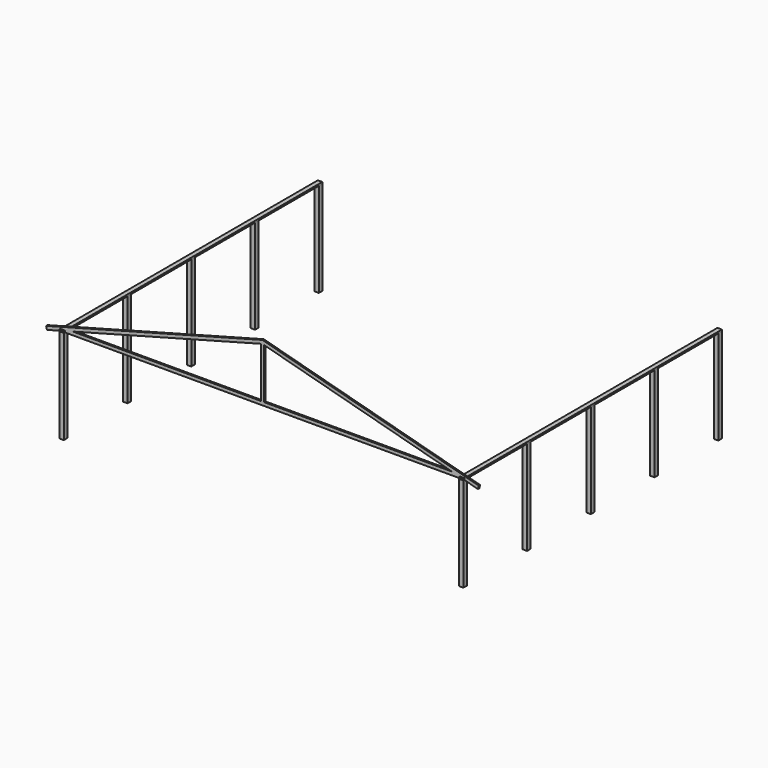
from build123d import *

# Parameters (mm, degrees)
F5_W      = 101.6
F5_H      = 101.6
F6_DEPTH  = 2133.6
F7_T      = -3.048
F7_2_T    = -3.048
F7_3_T    = -3.048
F7_4_T    = -3.048
F7_5_T    = -3.048
F11_DEPTH = 19.05
F10_W     = 76.2
F10_H     = 76.2
F12_DEPTH = 19.05
F13_T     = -3.048
F14_W     = 101.6
F14_H     = 38.1
F15_DEPTH = 7315.2
F16_T     = -3.048


with BuildPart() as f6:
    # F5 (on Top) → F6 (new body)
    with BuildSketch(Plane.XY):
        with Locations((-4521.2, 3606.8)):
            Rectangle(F5_W, F5_H)
    extrude(amount=F6_DEPTH)

    # F7
    f7_openings = [f6.faces().sort_by_distance(p)[0] for p in [
        (-4521.2, 3606.8, 2133.6),
        (-4521.2, 3606.8, 0),
    ]]
    offset(amount=F7_T, openings=f7_openings)


with BuildPart() as f6b:
    # F5 (on Top) → F6, piece 2 (new body)
    with BuildSketch(Plane.XY):
        with Locations((-4521.2, 1803.4)):
            Rectangle(F5_W, F5_H)
    extrude(amount=F6_DEPTH)

    # F7#2
    f7_2_openings = [f6b.faces().sort_by_distance(p)[0] for p in [
        (-4521.2, 1803.4, 2133.6),
        (-4521.2, 1803.4, 0),
    ]]
    offset(amount=F7_2_T, openings=f7_2_openings)


with BuildPart() as f6c:
    # F5 (on Top) → F6, piece 3 (new body)
    with BuildSketch(Plane.XY):
        with Locations((-4521.2, 0)):
            Rectangle(F5_W, F5_H)
    extrude(amount=F6_DEPTH)

    # F7#3
    f7_3_openings = [f6c.faces().sort_by_distance(p)[0] for p in [
        (-4521.2, 0, 2133.6),
        (-4521.2, 0, 0),
    ]]
    offset(amount=F7_3_T, openings=f7_3_openings)


with BuildPart() as f6d:
    # F5 (on Top) → F6, piece 4 (new body)
    with BuildSketch(Plane.XY):
        with Locations((-4521.2, -1803.4)):
            Rectangle(F5_W, F5_H)
    extrude(amount=F6_DEPTH)

    # F7#4
    f7_4_openings = [f6d.faces().sort_by_distance(p)[0] for p in [
        (-4521.2, -1803.4, 2133.6),
        (-4521.2, -1803.4, 0),
    ]]
    offset(amount=F7_4_T, openings=f7_4_openings)


with BuildPart() as f6e:
    # F5 (on Top) → F6, piece 5 (new body)
    with BuildSketch(Plane.XY):
        with Locations((-4521.2, -3606.8)):
            Rectangle(F5_W, F5_H)
    extrude(amount=F6_DEPTH)

    # F7#5
    f7_5_openings = [f6e.faces().sort_by_distance(p)[0] for p in [
        (-4521.2, -3606.8, 2133.6),
        (-4521.2, -3606.8, 0),
    ]]
    offset(amount=F7_5_T, openings=f7_5_openings)


with BuildPart() as f8_1:
    # F8: instance of F6c
    add(f6c.part.mirror(Plane.YZ))


with BuildPart() as f8_2:
    # F8: instance of F6d
    add(f6d.part.mirror(Plane.YZ))


with BuildPart() as f8_3:
    # F8: instance of F6e
    add(f6e.part.mirror(Plane.YZ))


with BuildPart() as f8_4:
    # F8: instance of F6b
    add(f6b.part.mirror(Plane.YZ))


with BuildPart() as f8_5:
    # F8: instance of F6
    add(f6.part.mirror(Plane.YZ))


with BuildPart() as f11:
    # F10 (on mid) → F11 (new body, symmetric)
    with BuildSketch(Plane.XZ.offset(3606.8)):
        Polygon((-4572, 2133.6), (-4572, 2209.8), (-4287.6177284633, 2209.8), (-38.1, 3348.4548435635), (0, 3358.6637077951), (38.1, 3348.4548435635), (4287.6177284633, 2209.8), (4572, 2209.8), (4572, 2133.6), (4876.8, 2051.929086147), (4896.5220112368, 2125.5326341102), (0, 3437.5517527423), (-4896.5220112368, 2125.5326341102), (-4876.8, 2051.929086147), align=None)
        Polygon((-4287.6177284633, 2209.8), (-4572, 2209.8), (-4572, 2133.6), align=None)
        Polygon((4572, 2209.8), (4287.6177284633, 2209.8), (4572, 2133.6), align=None)
    extrude(amount=F11_DEPTH, both=True)

    # F10 (on mid) → F12 (join, symmetric)
    with BuildSketch(Plane.XZ.offset(3606.8)):
        Polygon((-38.1, 2209.8), (-4287.6177284633, 2209.8), (-4572, 2133.6), (-38.1, 2133.6), align=None)
        Polygon((4287.6177284633, 2209.8), (38.1, 2209.8), (38.1, 2133.6), (4572, 2133.6), align=None)
        with Locations((0, 2171.7)):
            Rectangle(F10_W, F10_H)
        Polygon((-38.1, 3348.4548435635), (-38.1, 2209.8), (38.1, 2209.8), (38.1, 3348.4548435635), (0, 3358.6637077951), align=None)
    extrude(amount=F12_DEPTH, both=True)

    # F13
    f13_openings = [f11.faces().sort_by_distance(p)[0] for p in [
        (4886.661006, -3606.8, 2088.73086),
        (-4886.661006, -3606.8, 2088.73086),
    ]]
    offset(amount=F13_T, openings=f13_openings, kind=Kind.INTERSECTION)


with BuildPart() as f15:
    # F14 (on face) → F15 (new body, through all)
    with BuildSketch(Plane.XZ.offset(3657.6)):
        with Locations((4521.2, 2152.65)):
            Rectangle(F14_W, F14_H)
    extrude(amount=-F15_DEPTH)

    # F16
    f16_openings = [f15.faces().sort_by_distance(p)[0] for p in [
        (4521.2, 3657.6, 2152.65),
        (4521.2, -3657.6, 2152.65),
    ]]
    offset(amount=F16_T, openings=f16_openings)


with BuildPart() as f17_1:
    # F17: instance of F15
    add(f15.part.mirror(Plane.YZ))


solid = Compound([f6.part, f6b.part, f6c.part, f6d.part, f6e.part, f8_1.part, f8_2.part, f8_3.part, f8_4.part, f8_5.part, f11.part, f15.part, f17_1.part])
